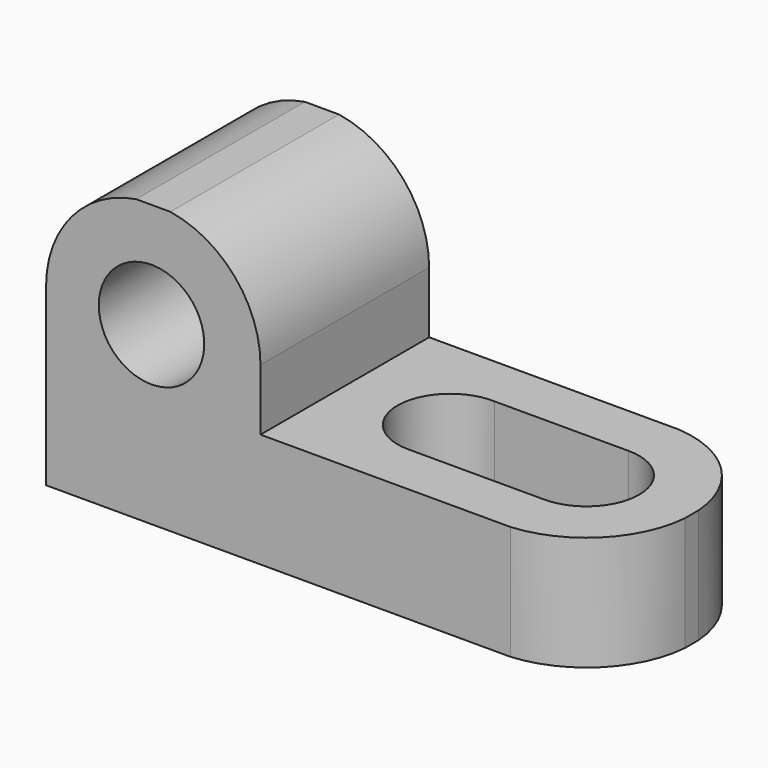
from build123d import *

# Parameters (mm, degrees)
F1_DEPTH = 25.4
F3_DEPTH = 50.8
F4_R     = 6.35
F5_DEPTH = 13.7715663219
F7_DEPTH = 13.7715663219
F9_DEPTH = 13.7715663219


with BuildPart() as f1:
    # F0 (on Front) → F1 (new body)
    with BuildSketch(Plane.XZ):
        Polygon((0, 33.8735803962), (0, 0), (67.6466450095, 0), (67.6466450095, 13.7705663219), (25.8323773742, 13.7705663219), (25.8323773742, 33.8735803962), align=None)
    extrude(amount=F1_DEPTH)

    # F2 (on face) → F3 (cut)
    with BuildSketch(Plane.XZ.offset(25.4)):
        with BuildLine():
            Line((0, 33.8735803962), (0, 21.1735803962))
            ThreePointArc((0, 21.1735803962), (3.0977100292, 29.5149442417), (10.8550581005, 33.8735803962))
            Line((10.8550581005, 33.8735803962), (0, 33.8735803962))
        make_face()
        with BuildLine():
            ThreePointArc((19.05, 21.1735803962), (12.7, 27.5235803962), (6.35, 21.1735803962))
            Line((6.35, 21.1735803962), (12.7, 21.1735803962))
            Line((12.7, 21.1735803962), (19.05, 21.1735803962))
        make_face()
        with BuildLine():
            Line((12.7, 21.1735803962), (6.35, 21.1735803962))
            ThreePointArc((6.35, 21.1735803962), (12.7, 14.8235803962), (19.05, 21.1735803962))
            Line((19.05, 21.1735803962), (12.7, 21.1735803962))
        make_face()
        with BuildLine():
            Line((25.8323773742, 33.8735803962), (14.9773192737, 33.8735803962))
            ThreePointArc((14.9773192737, 33.8735803962), (22.734667345, 29.5149442417), (25.8323773742, 21.1735803962))
            Line((25.8323773742, 21.1735803962), (25.8323773742, 33.8735803962))
        make_face()
    extrude(amount=-F3_DEPTH, mode=Mode.SUBTRACT)

    # F4 (on face) → F5 (cut, through all)
    with BuildSketch(Plane.XY.offset(13.7705663219)):
        with Locations((38.5323773742, -12.7)):
            Circle(F4_R)
        with Locations((54.9466450095, -12.7)):
            Circle(F4_R)
    extrude(amount=-F5_DEPTH, mode=Mode.SUBTRACT)

    # F6 (on face) → F7 (cut, through all)
    with BuildSketch(Plane.XY.offset(13.7705663219)):
        with BuildLine():
            Line((54.9441526312, -6.3500004891), (38.8158588696, -6.3563308534))
            ThreePointArc((38.8158588696, -6.3563308534), (43.121636982, -8.3112420605), (44.8823773742, -12.7))
            ThreePointArc((44.8823773742, -12.7), (43.0225055016, -17.1901279936), (38.5323775634, -19.05))
            Line((38.5323775634, -19.05), (54.9441526312, -19.0499995109))
            ThreePointArc((54.9441526312, -19.0499995109), (48.5966450095, -12.7), (54.9441526312, -6.3500004891))
        make_face()
    extrude(amount=-F7_DEPTH, mode=Mode.SUBTRACT)

    # F8 (on face) → F9 (cut, through all)
    with BuildSketch(Plane.XY.offset(13.7705663219)):
        with BuildLine():
            ThreePointArc((55.9713775557, 0), (63.9560866346, -3.6905583749), (67.6466450095, -11.6752674539))
            Line((67.6466450095, -11.6752674539), (67.6466450095, 0))
            Line((67.6466450095, 0), (55.9713775557, 0))
        make_face()
        with BuildLine():
            Line((67.6466450095, -25.4), (67.6466450095, -13.7247325461))
            ThreePointArc((67.6466450095, -13.7247325461), (63.9560866346, -21.7094416251), (55.9713775557, -25.4))
            Line((55.9713775557, -25.4), (67.6466450095, -25.4))
        make_face()
        with BuildLine():
            Line((53.9219124634, 0), (55.9713775557, 0))
            ThreePointArc((55.9713775557, 0), (54.9466450095, 0.0412745356), (53.9219124634, 0))
        make_face()
    extrude(amount=-F9_DEPTH, mode=Mode.SUBTRACT)


solid = f1.part
